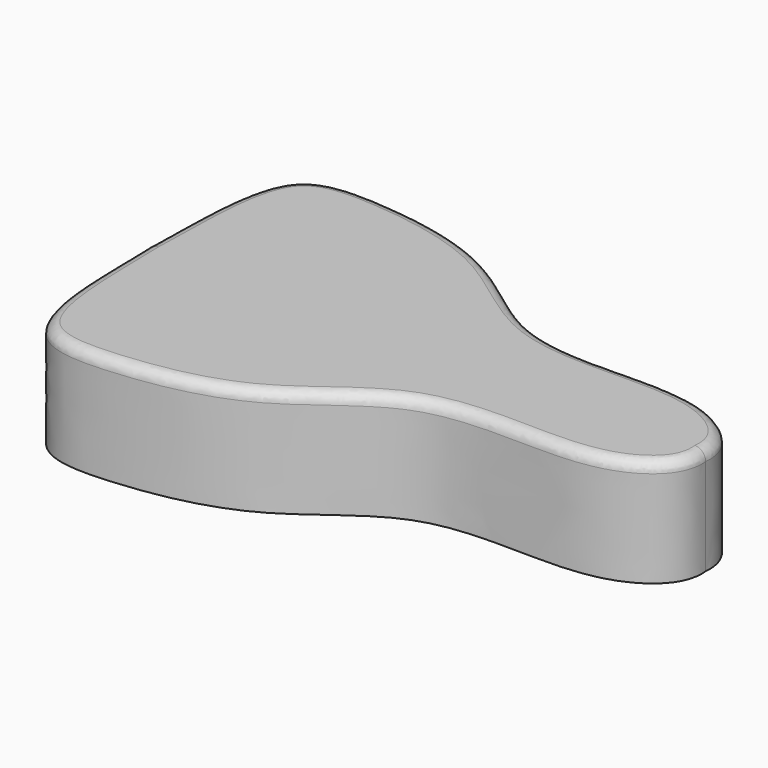
from build123d import *

# Parameters (mm, degrees)
F1_DEPTH = 50
F2_R     = 5


with BuildPart() as f1:
    # F0 (on Top) → F1 (new body)
    with BuildSketch(Plane.XY):
        with BuildLine():
            add(Edge.make_bspline(
                [(0, 0), (0.9194884541, 29.4002114479), (-1.1742920977, 80.0190413603), (47.790340102, 81.6056071987), (107.0005262857, 71.1421960021), (148.1857584102, 26.8220790626), (207.8726578314, 31.9044495279), (244.6728573572, 27.8856813881), (261.1163146223, 11.4676433787), (260, 0)],
                knots=[0, 0, 0, 0, 0.1745257722, 0.2983117542, 0.457177357, 0.6122981896, 0.7662906521, 0.8907051219, 1, 1, 1, 1], degree=3))
            Line((0, 0), (260, 0))
        make_face()
        with BuildLine():
            Line((260, 0), (0, 0))
            add(Edge.make_bspline(
                [(0, 0), (0.9194884541, -29.4002114479), (-1.1742920977, -80.0190413603), (47.790340102, -81.6056071987), (107.0005262857, -71.1421960021), (148.1857584102, -26.8220790626), (207.8726578314, -31.9044495279), (244.6728573572, -27.8856813881), (261.1163146223, -11.4676433787), (260, 0)],
                knots=[0, 0, 0, 0, 0.1745257722, 0.2983117542, 0.457177357, 0.6122981896, 0.7662906521, 0.8907051219, 1, 1, 1, 1], degree=3))
        make_face()
    extrude(amount=F1_DEPTH)

    # F2
    f2_edges = [f1.edges().sort_by_distance(p)[0] for p in [
        (107.976522, 62.92801, 50),
        (107.976522, -62.92801, 50),
    ]]
    fillet(f2_edges, radius=F2_R)


solid = f1.part
